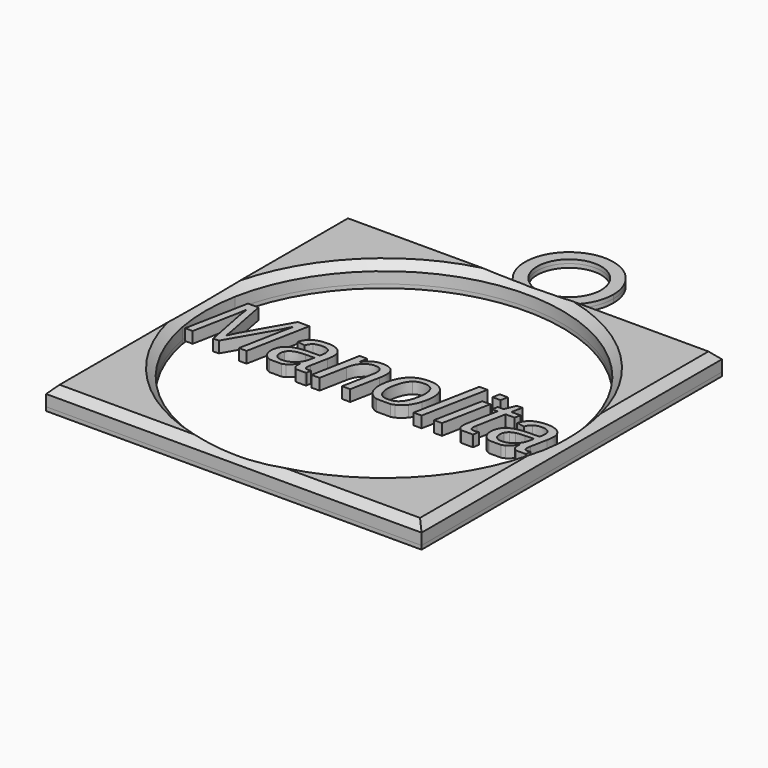
from build123d import *
from build123d import SkipClean  # not in build123d's __all__

# Parameters (mm, degrees)
F1_DEPTH     = 5
F0_R         = 8.5199022073
F2_DEPTH     = 1
F3_T1_DEPTH  = 58.7432495596
F3_T3_DEPTH  = 110.2867319519
F3_T5_DEPTH  = 110.2867319519
F3_T7_DEPTH  = 58.7432495596
F3_T10_ANGLE = 65.1626745713
F2_FACE_R    = 8.5199022073
F4_DEPTH     = 1
F5_DEPTH     = 3


# Not quite as in the source:
# - a fillet or chamfer that OpenCascade refuses, or shapes differently, is made with other operations: its cross-section is extruded or revolved along the edge and cut away or added
# - the program builds the solid bodies; features that only make, move or delete a surface that nothing else refers to are left out


with BuildPart() as f1:
    # F0 (on Top) → F1 (new body)
    with BuildSketch(Plane.XY):
        with BuildLine():
            Line((-50, 50), (-50, -50))
            Line((-50, -50), (50, -50))
            Line((50, -50), (50, 50))
            Line((50, 50), (1.5434823923, 50))
            ThreePointArc((1.5434823923, 50), (0, 49.898331828), (-1.5434823923, 50))
            Line((-1.5434823923, 50), (-50, 50))
        make_face()
        with BuildLine():
            ThreePointArc((46.6759421594, 8.8094508077), (47.2935368342, 4.4239545335), (47.5, 0))
            ThreePointArc((47.5, 0), (47.2935368342, -4.4239545335), (46.6759421594, -8.8094508077))
            ThreePointArc((46.6759421594, -8.8094508077), (0, -47.5), (-46.6759421594, -8.8094508077))
            ThreePointArc((-46.6759421594, -8.8094508077), (-47.5, 0), (-46.6759421594, 8.8094508077))
            ThreePointArc((-46.6759421594, 8.8094508077), (0, 47.5), (46.6759421594, 8.8094508077))
        make_face(mode=Mode.SUBTRACT)
    extrude(amount=F1_DEPTH)

    # F0 (on Top) → F2 (join)
    with BuildSketch(Plane.XY):
        with BuildLine():
            ThreePointArc((11.7670764853, 61.6654083133), (-7.7557015687, 70.5148818675), (-1.5434823923, 50))
            Line((-1.5434823923, 50), (1.5434823923, 50))
            ThreePointArc((1.5434823923, 50), (8.8494735542, 53.9097067445), (11.7670764853, 61.6654083133))
        make_face()
        with Locations((0, 61.6654083133)):
            Circle(F0_R, mode=Mode.SUBTRACT)
        with BuildLine():
            Line((-50, 50), (-50, -50))
            Line((-50, -50), (50, -50))
            Line((50, -50), (50, 50))
            Line((50, 50), (1.5434823923, 50))
            ThreePointArc((1.5434823923, 50), (0, 49.898331828), (-1.5434823923, 50))
            Line((-1.5434823923, 50), (-50, 50))
        make_face()
        with BuildLine():
            ThreePointArc((46.6759421594, 8.8094508077), (47.2935368342, 4.4239545335), (47.5, 0))
            ThreePointArc((47.5, 0), (47.2935368342, -4.4239545335), (46.6759421594, -8.8094508077))
            ThreePointArc((46.6759421594, -8.8094508077), (0, -47.5), (-46.6759421594, -8.8094508077))
            ThreePointArc((-46.6759421594, -8.8094508077), (-47.5, 0), (-46.6759421594, 8.8094508077))
            ThreePointArc((-46.6759421594, 8.8094508077), (0, 47.5), (46.6759421594, 8.8094508077))
        make_face(mode=Mode.SUBTRACT)
        with BuildLine():
            Line((1.5434823923, 50), (-1.5434823923, 50))
            ThreePointArc((-1.5434823923, 50), (0, 49.898331828), (1.5434823923, 50))
        make_face()
    extrude(amount=F2_DEPTH)

    # F3: chamfer of 2 on 7 edges, made by hand

    # F3_s2 → F3_t1 (cut)
    with BuildSketch(Plane.YZ.offset(-55.1433659759)):
        Polygon((48, 5), (50, 3), (50, 5), align=None)
    extrude(amount=F3_T1_DEPTH, mode=Mode.SUBTRACT)

    # F3_s4 → F3_t3 (cut)
    with BuildSketch(Plane.XZ.offset(-55.1433659759)):
        Polygon((-48, 5), (-50, 3), (-50, 5), align=None)
        Polygon((48, 5), (50, 3), (50, 5), align=None)
    extrude(amount=F3_T3_DEPTH, mode=Mode.SUBTRACT)

    # F3_s6 → F3_t5 (cut)
    with BuildSketch(Plane.YZ.offset(-55.1433659759)):
        Polygon((-48, 5), (-50, 3), (-50, 5), align=None)
    extrude(amount=F3_T5_DEPTH, mode=Mode.SUBTRACT)

    # F3_s8 → F3_t7 (cut)
    with BuildSketch(Plane.YZ.offset(-3.5998835836)):
        Polygon((48, 5), (50, 3), (50, 5), align=None)
    extrude(amount=F3_T7_DEPTH, mode=Mode.SUBTRACT)

    # F3_s9 → F3_t10 (revolve, cut)
    with BuildSketch(Plane(origin=(27.9808033762, 17.881631304, 0), x_dir=(0, 0, 1), z_dir=(0.8426278439, 0.5384963479, 0))):
        Polygon((3, -40.1939135628), (5, -38.1939135628), (5, -40.1939135628), align=None)
    revolve(axis=Axis((0, 61.6654083133, 5), (0, 0, -1)), revolution_arc=F3_T10_ANGLE, mode=Mode.SUBTRACT)

    # F3_s11 → F3_t12 (revolve, cut)
    with BuildSketch(Plane(origin=(0, 0, 0), x_dir=(0, 0, 1), z_dir=(0.1854621223, 0.9826514139, 0))):
        Polygon((5, -49.5), (3, -47.5), (5, -47.5), align=None)
    revolve(axis=Axis((0, 0, 5), (0, 0, 1)), mode=Mode.SUBTRACT)

    # F0 (on Top) + F2_face (on face) → F4 (join)
    with BuildSketch(Plane.XY):
        with BuildLine():
            Line((-50, 50), (-50, -50))
            Line((-50, -50), (50, -50))
            Line((50, -50), (50, 50))
            Line((50, 50), (1.5434823923, 50))
            ThreePointArc((1.5434823923, 50), (0, 49.898331828), (-1.5434823923, 50))
            Line((-1.5434823923, 50), (-50, 50))
        make_face()
        with BuildLine():
            ThreePointArc((46.6759421594, 8.8094508077), (47.2935368342, 4.4239545335), (47.5, 0))
            ThreePointArc((47.5, 0), (47.2935368342, -4.4239545335), (46.6759421594, -8.8094508077))
            ThreePointArc((46.6759421594, -8.8094508077), (0, -47.5), (-46.6759421594, -8.8094508077))
            ThreePointArc((-46.6759421594, -8.8094508077), (-47.5, 0), (-46.6759421594, 8.8094508077))
            ThreePointArc((-46.6759421594, 8.8094508077), (0, 47.5), (46.6759421594, 8.8094508077))
        make_face(mode=Mode.SUBTRACT)
        with BuildLine():
            ThreePointArc((11.7670764853, 61.6654083133), (-7.7557015687, 70.5148818675), (-1.5434823923, 50))
            Line((-1.5434823923, 50), (1.5434823923, 50))
            ThreePointArc((1.5434823923, 50), (8.8494735542, 53.9097067445), (11.7670764853, 61.6654083133))
        make_face()
        with Locations((0, 61.6654083133)):
            Circle(F0_R, mode=Mode.SUBTRACT)
        with BuildLine():
            Line((1.5434823923, 50), (-1.5434823923, 50))
            ThreePointArc((-1.5434823923, 50), (0, 49.898331828), (1.5434823923, 50))
        make_face()
    with BuildSketch(Plane(origin=(0, 61.6654083133, 1), x_dir=(1, 0, 0), z_dir=(0, 0, 1))):
        with BuildLine():
            ThreePointArc((-1.5434823923, -11.6654083133), (0, -11.7670764853), (1.5434823923, -11.6654083133))
            ThreePointArc((1.5434823923, -11.6654083133), (0, 11.7670764853), (-1.5434823923, -11.6654083133))
        make_face()
        Circle(F2_FACE_R, mode=Mode.SUBTRACT)
    with SkipClean():  # cleaning this boolean's faces spoils the solid; the shape is the same uncleaned
        extrude(amount=-F4_DEPTH)


with BuildPart() as f5:
    # F0 (on Top) → F5 (new body)
    with BuildSketch(Plane.XY):
        Polygon((25.5470249877, 6.8670892581), (25.9333310952, 8.8094508077), (23.7808877048, 8.8094508077), (23.3981919348, 6.8670892581), align=None)
        with BuildLine():
            Line((42.3061471078, -8.8094508077), (44.4772175829, -8.8094508077))
            add(Edge.make_bspline(
                [(44.8100515369, -8.7368034269), (44.6425976503, -8.7774475742), (44.4772175829, -8.8094508077)],
                knots=[0, 0, 0, 0.2125992126, 0.2125992126, 0.2125992126], degree=2))
            Line((44.8100515369, -8.7368034269), (44.9782875766, -7.3985622018))
            add(Edge.make_bspline(
                [(44.2594608614, -7.4826802217), (44.5844623018, -7.4826802217), (44.9782875766, -7.3985622018)],
                knots=[0, 0, 0, 1, 1, 1], degree=2))
            add(Edge.make_bspline(
                [(43.292103633, -6.6109116521), (43.292103633, -7.4826802217), (44.2594608614, -7.4826802217)],
                knots=[0, 0, 0, 1, 1, 1], degree=2))
            add(Edge.make_bspline(
                [(43.4221042091, -5.5594364038), (43.292103633, -6.1329683575), (43.292103633, -6.6109116521)],
                knots=[0, 0, 0, 1, 1, 1], degree=2))
            Line((43.4221042091, -5.5594364038), (44.3091669641, -1.0438281556))
            add(Edge.make_bspline(
                [(44.5347561992, 0.8335331059), (44.5347561992, 0.0688238344), (44.3091669641, -1.0438281556)],
                knots=[0, 0, 0, 1, 1, 1], degree=2))
            add(Edge.make_bspline(
                [(43.345633282, 3.4029562582), (44.5347561992, 2.4470696688), (44.5347561992, 0.8335331059)],
                knots=[0, 0, 0, 1, 1, 1], degree=2))
            add(Edge.make_bspline(
                [(40.1147366099, 4.3588428476), (42.1565103648, 4.3588428476), (43.345633282, 3.4029562582)],
                knots=[0, 0, 0, 1, 1, 1], degree=2))
            add(Edge.make_bspline(
                [(36.5339854461, 3.5635452052), (37.8664913517, 4.3588428476), (40.1147366099, 4.3588428476)],
                knots=[0, 0, 0, 1, 1, 1], degree=2))
            add(Edge.make_bspline(
                [(34.6661830504, 1.0132397847), (35.2014795405, 2.7682475628), (36.5339854461, 3.5635452052)],
                knots=[0, 0, 0, 1, 1, 1], degree=2))
            Line((34.6661830504, 1.0132397847), (36.7920748252, 0.6652970662))
            add(Edge.make_bspline(
                [(37.8435500735, 2.213833341), (37.1132527192, 1.7053016755), (36.7920748252, 0.6652970662)],
                knots=[0, 0, 0, 1, 1, 1], degree=2))
            add(Edge.make_bspline(
                [(39.9962066728, 2.7223650066), (38.5738474278, 2.7223650066), (37.8435500735, 2.213833341)],
                knots=[0, 0, 0, 1, 1, 1], degree=2))
            add(Edge.make_bspline(
                [(41.7512144509, 2.2023627019), (41.1165057556, 2.7223650066), (39.9962066728, 2.7223650066)],
                knots=[0, 0, 0, 1, 1, 1], degree=2))
            add(Edge.make_bspline(
                [(42.3859231463, 0.5926496854), (42.3859231463, 1.6823603973), (41.7512144509, 2.2023627019)],
                knots=[0, 0, 0, 1, 1, 1], degree=2))
            add(Edge.make_bspline(
                [(42.1565103648, -0.9214746722), (42.3859231463, 0.2485305132), (42.3859231463, 0.5926496854)],
                knots=[0, 0, 0, 1, 1, 1], degree=2))
            Line((42.1565103648, -0.9214746722), (39.3844392556, -0.9597101357))
            add(Edge.make_bspline(
                [(34.3373580637, -2.1411859602), (35.9203062557, -1.005592692), (39.3844392556, -0.9597101357)],
                knots=[0, 0, 0, 1, 1, 1], degree=2))
            add(Edge.make_bspline(
                [(32.7544098717, -5.486789023), (32.7544098717, -3.2767792284), (34.3373580637, -2.1411859602)],
                knots=[0, 0, 0, 1, 1, 1], degree=2))
            add(Edge.make_bspline(
                [(33.8001498004, -8.0447415362), (32.7544098717, -7.0391488442), (32.7544098717, -5.486789023)],
                knots=[0, 0, 0, 1, 1, 1], degree=2))
            add(Edge.make_bspline(
                [(35.0309562259, -8.8094508077), (34.3340710978, -8.558164941), (33.8001498004, -8.0447415362)],
                knots=[0.4894320446, 0.4894320446, 0.4894320446, 1, 1, 1], degree=2))
            Line((35.0309562259, -8.8094508077), (38.2424706133, -8.8094508077))
            add(Edge.make_bspline(
                [(39.0862026397, -8.4462139038), (38.6944582041, -8.6688600218), (38.2424706133, -8.8094508077)],
                knots=[0, 0, 0, 0.3685459817, 0.3685459817, 0.3685459817], degree=2))
            add(Edge.make_bspline(
                [(41.1432705801, -6.3356163144), (40.1491485271, -7.8420935793), (39.0862026397, -8.4462139038)],
                knots=[0, 0, 0, 1, 1, 1], degree=2))
            Line((41.1432705801, -6.3356163144), (41.2120944145, -6.3356163144))
            Line((41.2120944145, -6.3356163144), (41.1547412191, -7.1003255859))
            add(Edge.make_bspline(
                [(41.6613611115, -8.4691551819), (41.1547412191, -8.010329619), (41.1547412191, -7.1003255859)],
                knots=[0, 0, 0, 1, 1, 1], degree=2))
            add(Edge.make_bspline(
                [(42.3061471078, -8.8094508077), (41.9104838328, -8.6947757596), (41.6613611115, -8.4691551819)],
                knots=[0.5082650227, 0.5082650227, 0.5082650227, 1, 1, 1], degree=2))
        make_face()
        with BuildLine():
            Line((39.4914985536, -2.4508932152), (41.869744388, -2.4050106589))
            Line((41.869744388, -2.4050106589), (41.548566494, -3.9000172847))
            add(Edge.make_bspline(
                [(40.7475335321, -5.6187013724), (41.3573891761, -4.8176684105), (41.548566494, -3.9000172847)],
                knots=[0, 0, 0, 1, 1, 1], degree=2))
            add(Edge.make_bspline(
                [(39.20664435, -6.9148835876), (40.137677888, -6.4197343343), (40.7475335321, -5.6187013724)],
                knots=[0, 0, 0, 1, 1, 1], degree=2))
            add(Edge.make_bspline(
                [(37.1132527192, -7.4100328409), (38.2756108119, -7.4100328409), (39.20664435, -6.9148835876)],
                knots=[0, 0, 0, 1, 1, 1], degree=2))
            add(Edge.make_bspline(
                [(35.6163343203, -6.8498832995), (36.1956015934, -7.4100328409), (37.1132527192, -7.4100328409)],
                knots=[0, 0, 0, 1, 1, 1], degree=2))
            add(Edge.make_bspline(
                [(35.0370670471, -5.3912003641), (35.0370670471, -6.2897337581), (35.6163343203, -6.8498832995)],
                knots=[0, 0, 0, 1, 1, 1], degree=2))
            add(Edge.make_bspline(
                [(35.2932446531, -4.1313418393), (35.0370670471, -4.6494323707), (35.0370670471, -5.3912003641)],
                knots=[0, 0, 0, 1, 1, 1], degree=2))
            add(Edge.make_bspline(
                [(35.9967771828, -3.2710439089), (35.549422259, -3.6132513079), (35.2932446531, -4.1313418393)],
                knots=[0, 0, 0, 1, 1, 1], degree=2))
            add(Edge.make_bspline(
                [(37.2566357076, -2.7089825943), (36.4441321067, -2.9288365099), (35.9967771828, -3.2710439089)],
                knots=[0, 0, 0, 1, 1, 1], degree=2))
            add(Edge.make_bspline(
                [(39.4914985536, -2.4508932152), (38.0691393086, -2.4891286787), (37.2566357076, -2.7089825943)],
                knots=[0, 0, 0, 1, 1, 1], degree=2))
        make_face(mode=Mode.SUBTRACT)
        Polygon((20.4967286534, 8.8094508077), (18.3441462497, 8.8094508077), (14.9252132066, -8.8094508077), (17.0663991668, -8.8094508077), align=None)
        with BuildLine():
            Line((-42.661218484, 8.0256238044), (-45.922703527, -8.8094508077))
            Line((-45.922703527, -8.8094508077), (-43.8924004111, -8.8094508077))
            add(Edge.make_bspline(
                [(-41.5007721645, 3.6228101737), (-41.7512144509, 2.0991269503), (-43.8924004111, -8.8094508077)],
                knots=[0, 0, 0, 1, 1, 1], degree=2))
            add(Edge.make_bspline(
                [(-41.1432705801, 5.8653201124), (-41.2503298781, 5.1464933972), (-41.5007721645, 3.6228101737)],
                knots=[0, 0, 0, 1, 1, 1], degree=2))
            add(Edge.make_bspline(
                [(-40.6538566463, 2.5197170496), (-40.7265040271, 2.8638362218), (-41.1432705801, 5.8653201124)],
                knots=[0, 0, 0, 1, 1, 1], degree=2))
            Line((-40.6538566463, 2.5197170496), (-38.4438468517, -8.8094508077))
            Line((-38.4438468517, -8.8094508077), (-36.9603108649, -8.8094508077))
            Line((-36.9603108649, -8.8094508077), (-30.4143995009, 2.5197170496))
            add(Edge.make_bspline(
                [(-28.6823330009, 5.8653201124), (-29.7682201664, 3.6056042151), (-30.4143995009, 2.5197170496)],
                knots=[0, 0, 0, 1, 1, 1], degree=2))
            add(Edge.make_bspline(
                [(-29.4585129115, 2.2788336291), (-29.0264521731, 4.4888434237), (-28.6823330009, 5.8653201124)],
                knots=[0, 0, 0, 1, 1, 1], degree=2))
            Line((-29.4585129115, 2.2788336291), (-31.6073459644, -8.8094508077))
            Line((-31.6073459644, -8.8094508077), (-29.5541015704, -8.8094508077))
            Line((-29.5541015704, -8.8094508077), (-26.2926165275, 8.0256238044))
            Line((-26.2926165275, 8.0256238044), (-29.3514536135, 8.0256238044))
            Line((-29.3514536135, 8.0256238044), (-35.9585417193, -3.5520745661))
            Line((-35.9585417193, -3.5520745661), (-37.2011942855, -6.0985564402))
            add(Edge.make_bspline(
                [(-37.5835489212, -3.6476632251), (-37.4879602623, -4.1141358807), (-37.2011942855, -6.0985564402)],
                knots=[0, 0, 0, 1, 1, 1], degree=2))
            Line((-37.5835489212, -3.6476632251), (-39.8394412721, 8.0256238044))
            Line((-39.8394412721, 8.0256238044), (-42.661218484, 8.0256238044))
        make_face()
        with BuildLine():
            Line((5.021726883, -8.8094508077), (8.7657562591, -8.8094508077))
            add(Edge.make_bspline(
                [(9.7309254799, -8.4691551819), (9.2712635293, -8.6761733048), (8.7657562591, -8.8094508077)],
                knots=[0, 0, 0, 0.3562036935, 0.3562036935, 0.3562036935], degree=2))
            add(Edge.make_bspline(
                [(11.9103469037, -6.7237062697), (11.0213723755, -7.8879761356), (9.7309254799, -8.4691551819)],
                knots=[0, 0, 0, 1, 1, 1], degree=2))
            add(Edge.make_bspline(
                [(13.2772647265, -3.8808995529), (12.7993214318, -5.5594364038), (11.9103469037, -6.7237062697)],
                knots=[0, 0, 0, 1, 1, 1], degree=2))
            add(Edge.make_bspline(
                [(13.7552080212, -0.6500028808), (13.7552080212, -2.2023627019), (13.2772647265, -3.8808995529)],
                knots=[0, 0, 0, 1, 1, 1], degree=2))
            add(Edge.make_bspline(
                [(12.4303492083, 3.037807581), (13.7552080212, 1.7282429536), (13.7552080212, -0.6500028808)],
                knots=[0, 0, 0, 1, 1, 1], degree=2))
            add(Edge.make_bspline(
                [(8.5934204385, 4.3473722085), (11.1054903954, 4.3473722085), (12.4303492083, 3.037807581)],
                knots=[0, 0, 0, 1, 1, 1], degree=2))
            add(Edge.make_bspline(
                [(4.9247277085, 3.3781032069), (6.406351922, 4.3473722085), (8.5934204385, 4.3473722085)],
                knots=[0, 0, 0, 1, 1, 1], degree=2))
            add(Edge.make_bspline(
                [(2.6076586158, 0.5219140778), (3.4431034949, 2.4088342052), (4.9247277085, 3.3781032069)],
                knots=[0, 0, 0, 1, 1, 1], degree=2))
            add(Edge.make_bspline(
                [(1.7225076341, -3.8044286257), (1.7722137367, -1.3650060496), (2.6076586158, 0.5219140778)],
                knots=[0, 0, 0, 1, 1, 1], degree=2))
            add(Edge.make_bspline(
                [(3.0856019105, -7.6394456223), (1.7225076341, -6.2285570164), (1.7225076341, -3.8044286257)],
                knots=[0, 0, 0, 1, 1, 1], degree=2))
            add(Edge.make_bspline(
                [(5.021726883, -8.8094508077), (3.8854698095, -8.4673593803), (3.0856019105, -7.6394456223)],
                knots=[0.4131969353, 0.4131969353, 0.4131969353, 1, 1, 1], degree=2))
        make_face()
        with BuildLine():
            add(Edge.make_bspline(
                [(11.5337275874, -0.6500028808), (11.5337275874, 2.7682475628), (8.5704791604, 2.7682475628)],
                knots=[0, 0, 0, 1, 1, 1], degree=2))
            add(Edge.make_bspline(
                [(11.1207845808, -3.5157508757), (11.4725508457, -2.1526565993), (11.5337275874, -0.6500028808)],
                knots=[0, 0, 0, 1, 1, 1], degree=2))
            add(Edge.make_bspline(
                [(10.2069570014, -5.7563490412), (10.7690183159, -4.8788451522), (11.1207845808, -3.5157508757)],
                knots=[0, 0, 0, 1, 1, 1], degree=2))
            add(Edge.make_bspline(
                [(8.8993041471, -7.0467959369), (9.6448956868, -6.6338529303), (10.2069570014, -5.7563490412)],
                knots=[0, 0, 0, 1, 1, 1], degree=2))
            add(Edge.make_bspline(
                [(6.9225306803, -7.4597389435), (8.1537126074, -7.4597389435), (8.8993041471, -7.0467959369)],
                knots=[0, 0, 0, 1, 1, 1], degree=2))
            add(Edge.make_bspline(
                [(4.7010502466, -6.5325289518), (5.4657595181, -7.4597389435), (6.9225306803, -7.4597389435)],
                knots=[0, 0, 0, 1, 1, 1], degree=2))
            add(Edge.make_bspline(
                [(3.9363409751, -3.8388405429), (3.9363409751, -5.6053189601), (4.7010502466, -6.5325289518)],
                knots=[0, 0, 0, 1, 1, 1], degree=2))
            add(Edge.make_bspline(
                [(4.4735492383, -0.5754437268), (3.9363409751, -2.2597158973), (3.9363409751, -3.8388405429)],
                knots=[0, 0, 0, 1, 1, 1], degree=2))
            add(Edge.make_bspline(
                [(5.9838500495, 1.9385380033), (5.0107575015, 1.1088284437), (4.4735492383, -0.5754437268)],
                knots=[0, 0, 0, 1, 1, 1], degree=2))
            add(Edge.make_bspline(
                [(8.5704791604, 2.7682475628), (6.9569425975, 2.7682475628), (5.9838500495, 1.9385380033)],
                knots=[0, 0, 0, 1, 1, 1], degree=2))
        make_face(mode=Mode.SUBTRACT)
        Polygon((22.8705425375, 4.117959427), (20.362296127, -8.8094508077), (22.5034820872, -8.8094508077), (25.0231991368, 4.117959427), align=None)
        with BuildLine():
            Line((27.5877950428, -8.8094508077), (30.5493130455, -8.8094508077))
            add(Edge.make_bspline(
                [(30.758518673, -8.7597447051), (30.652735788, -8.785762502), (30.5493130455, -8.8094508077)],
                knots=[0, 0, 0, 0.089534532, 0.089534532, 0.089534532], degree=2))
            Line((30.758518673, -8.7597447051), (30.9841079081, -7.1729729667))
            add(Edge.make_bspline(
                [(29.7911614446, -7.3412090064), (30.2920460174, -7.3412090064), (30.9841079081, -7.1729729667)],
                knots=[0, 0, 0, 1, 1, 1], degree=2))
            add(Edge.make_bspline(
                [(28.7167449181, -6.2897337581), (28.7167449181, -7.3412090064), (29.7911614446, -7.3412090064)],
                knots=[0, 0, 0, 1, 1, 1], degree=2))
            add(Edge.make_bspline(
                [(28.8582161334, -5.1541404899), (28.7167449181, -5.8691436588), (28.7167449181, -6.2897337581)],
                knots=[0, 0, 0, 1, 1, 1], degree=2))
            Line((28.8582161334, -5.1541404899), (30.3532227591, 2.5541289668))
            Line((30.3532227591, 2.5541289668), (32.7429392326, 2.5541289668))
            Line((32.7429392326, 2.5541289668), (33.0526464876, 4.117959427))
            Line((33.0526464876, 4.117959427), (30.6629300141, 4.117959427))
            Line((30.6629300141, 4.117959427), (31.2249913287, 7.0123840197))
            Line((31.2249913287, 7.0123840197), (29.7911614446, 7.0123840197))
            Line((29.7911614446, 7.0123840197), (28.5370382393, 4.117959427))
            Line((28.5370382393, 4.117959427), (27.0190903354, 4.117959427))
            Line((27.0190903354, 4.117959427), (26.7093830804, 2.5541289668))
            Line((26.7093830804, 2.5541289668), (28.2005661599, 2.5541289668))
            Line((28.2005661599, 2.5541289668), (26.6979124414, -5.272670427))
            add(Edge.make_bspline(
                [(26.5182057626, -6.8250302482), (26.5182057626, -6.1673802747), (26.6979124414, -5.272670427)],
                knots=[0, 0, 0, 1, 1, 1], degree=2))
            add(Edge.make_bspline(
                [(27.0974730357, -8.4404785842), (26.5182057626, -7.8306229402), (26.5182057626, -6.8250302482)],
                knots=[0, 0, 0, 1, 1, 1], degree=2))
            add(Edge.make_bspline(
                [(27.5877950428, -8.8094508077), (27.3126836962, -8.667053504), (27.0974730357, -8.4404785842)],
                knots=[0.6284777848, 0.6284777848, 0.6284777848, 1, 1, 1], degree=2))
        make_face()
        with BuildLine():
            Line((-4.1160476539, -8.8094508077), (-1.9557439619, -8.8094508077))
            Line((-1.9557439619, -8.8094508077), (-0.4377960579, -1.005592692))
            add(Edge.make_bspline(
                [(-0.1854419983, 0.952063043), (-0.1854419983, 0.1873537715), (-0.4377960579, -1.005592692)],
                knots=[0, 0, 0, 1, 1, 1], degree=2))
            add(Edge.make_bspline(
                [(-1.0763282996, 3.4736918658), (-0.1854419983, 2.6000115231), (-0.1854419983, 0.952063043)],
                knots=[0, 0, 0, 1, 1, 1], degree=2))
            add(Edge.make_bspline(
                [(-3.7336930181, 4.3473722085), (-1.9672146009, 4.3473722085), (-1.0763282996, 3.4736918658)],
                knots=[0, 0, 0, 1, 1, 1], degree=2))
            add(Edge.make_bspline(
                [(-6.1081153061, 3.8158992648), (-5.1101697068, 4.3473722085), (-3.7336930181, 4.3473722085)],
                knots=[0, 0, 0, 1, 1, 1], degree=2))
            add(Edge.make_bspline(
                [(-8.096359412, 1.9079496324), (-7.1060609054, 3.2844263211), (-6.1081153061, 3.8158992648)],
                knots=[0, 0, 0, 1, 1, 1], degree=2))
            Line((-8.096359412, 1.9079496324), (-8.1307713293, 1.9079496324))
            add(Edge.make_bspline(
                [(-7.9223880528, 3.1926612085), (-8.0466533094, 2.3973635662), (-8.1307713293, 1.9079496324)],
                knots=[0, 0, 0, 1, 1, 1], degree=2))
            add(Edge.make_bspline(
                [(-7.7981227962, 4.117959427), (-7.7981227962, 3.9879588509), (-7.9223880528, 3.1926612085)],
                knots=[0, 0, 0, 1, 1, 1], degree=2))
            Line((-7.7981227962, 4.117959427), (-9.828425912, 4.117959427))
            add(Edge.make_bspline(
                [(-10.2948985676, 1.3573589569), (-10.0540151471, 2.4929522251), (-9.828425912, 4.117959427)],
                knots=[0, 0, 0, 1, 1, 1], degree=2))
            Line((-10.2948985676, 1.3573589569), (-12.2793191272, -8.8094508077))
            Line((-12.2793191272, -8.8094508077), (-10.1266625279, -8.8094508077))
            Line((-10.1266625279, -8.8094508077), (-8.715773922, -1.5676540066))
            add(Edge.make_bspline(
                [(-7.186355379, 1.5370656357), (-8.3334192862, 0.3900017285), (-8.715773922, -1.5676540066)],
                knots=[0, 0, 0, 1, 1, 1], degree=2))
            add(Edge.make_bspline(
                [(-4.5366377532, 2.684129543), (-6.0392914717, 2.684129543), (-7.186355379, 1.5370656357)],
                knots=[0, 0, 0, 1, 1, 1], degree=2))
            add(Edge.make_bspline(
                [(-2.395451793, 0.6882383444), (-2.395451793, 2.684129543), (-4.5366377532, 2.684129543)],
                knots=[0, 0, 0, 1, 1, 1], degree=2))
            add(Edge.make_bspline(
                [(-2.6133939354, -1.101181351), (-2.395451793, -0.0497061026), (-2.395451793, 0.6882383444)],
                knots=[0, 0, 0, 1, 1, 1], degree=2))
            Line((-2.6133939354, -1.101181351), (-4.1160476539, -8.8094508077))
        make_face()
        with BuildLine():
            add(Edge.make_bspline(
                [(-23.4654794978, -8.8094508077), (-24.1623646258, -8.558164941), (-24.6962859232, -8.0447415362)],
                knots=[0.4894320446, 0.4894320446, 0.4894320446, 1, 1, 1], degree=2))
            Line((-23.4654794978, -8.8094508077), (-20.2539651103, -8.8094508077))
            add(Edge.make_bspline(
                [(-19.4102330839, -8.4462139038), (-19.8019775195, -8.6688600218), (-20.2539651103, -8.8094508077)],
                knots=[0, 0, 0, 0.3685459817, 0.3685459817, 0.3685459817], degree=2))
            add(Edge.make_bspline(
                [(-17.3531651436, -6.3356163144), (-18.3472871965, -7.8420935793), (-19.4102330839, -8.4462139038)],
                knots=[0, 0, 0, 1, 1, 1], degree=2))
            Line((-17.3531651436, -6.3356163144), (-17.2843413092, -6.3356163144))
            Line((-17.2843413092, -6.3356163144), (-17.3416945045, -7.1003255859))
            add(Edge.make_bspline(
                [(-16.8350746121, -8.4691551819), (-17.3416945045, -8.010329619), (-17.3416945045, -7.1003255859)],
                knots=[0, 0, 0, 1, 1, 1], degree=2))
            add(Edge.make_bspline(
                [(-16.1902886159, -8.8094508077), (-16.5859518909, -8.6947757596), (-16.8350746121, -8.4691551819)],
                knots=[0.5082650227, 0.5082650227, 0.5082650227, 1, 1, 1], degree=2))
            Line((-16.1902886159, -8.8094508077), (-14.0192181408, -8.8094508077))
            add(Edge.make_bspline(
                [(-13.6863841867, -8.7368034269), (-13.8538380734, -8.7774475742), (-14.0192181408, -8.8094508077)],
                knots=[0, 0, 0, 0.2125992126, 0.2125992126, 0.2125992126], degree=2))
            Line((-13.6863841867, -8.7368034269), (-13.518148147, -7.3985622018))
            add(Edge.make_bspline(
                [(-14.2369748622, -7.4826802217), (-13.9119734218, -7.4826802217), (-13.518148147, -7.3985622018)],
                knots=[0, 0, 0, 1, 1, 1], degree=2))
            add(Edge.make_bspline(
                [(-15.2043320907, -6.6109116521), (-15.2043320907, -7.4826802217), (-14.2369748622, -7.4826802217)],
                knots=[0, 0, 0, 1, 1, 1], degree=2))
            add(Edge.make_bspline(
                [(-15.0743315145, -5.5594364038), (-15.2043320907, -6.1329683575), (-15.2043320907, -6.6109116521)],
                knots=[0, 0, 0, 1, 1, 1], degree=2))
            Line((-15.0743315145, -5.5594364038), (-14.1872687596, -1.0438281556))
            add(Edge.make_bspline(
                [(-13.9616795245, 0.8335331059), (-13.9616795245, 0.0688238344), (-14.1872687596, -1.0438281556)],
                knots=[0, 0, 0, 1, 1, 1], degree=2))
            add(Edge.make_bspline(
                [(-15.1508024417, 3.4029562582), (-13.9616795245, 2.4470696688), (-13.9616795245, 0.8335331059)],
                knots=[0, 0, 0, 1, 1, 1], degree=2))
            add(Edge.make_bspline(
                [(-18.3816991138, 4.3588428476), (-16.3399253588, 4.3588428476), (-15.1508024417, 3.4029562582)],
                knots=[0, 0, 0, 1, 1, 1], degree=2))
            add(Edge.make_bspline(
                [(-21.9624502776, 3.5635452052), (-20.629944372, 4.3588428476), (-18.3816991138, 4.3588428476)],
                knots=[0, 0, 0, 1, 1, 1], degree=2))
            add(Edge.make_bspline(
                [(-23.8302526732, 1.0132397847), (-23.2949561832, 2.7682475628), (-21.9624502776, 3.5635452052)],
                knots=[0, 0, 0, 1, 1, 1], degree=2))
            Line((-23.8302526732, 1.0132397847), (-21.7043608984, 0.6652970662))
            add(Edge.make_bspline(
                [(-20.6528856501, 2.213833341), (-21.3831830044, 1.7053016755), (-21.7043608984, 0.6652970662)],
                knots=[0, 0, 0, 1, 1, 1], degree=2))
            add(Edge.make_bspline(
                [(-18.5002290508, 2.7223650066), (-19.9225882958, 2.7223650066), (-20.6528856501, 2.213833341)],
                knots=[0, 0, 0, 1, 1, 1], degree=2))
            add(Edge.make_bspline(
                [(-16.7452212727, 2.2023627019), (-17.3799299681, 2.7223650066), (-18.5002290508, 2.7223650066)],
                knots=[0, 0, 0, 1, 1, 1], degree=2))
            add(Edge.make_bspline(
                [(-16.1105125774, 0.5926496854), (-16.1105125774, 1.6823603973), (-16.7452212727, 2.2023627019)],
                knots=[0, 0, 0, 1, 1, 1], degree=2))
            add(Edge.make_bspline(
                [(-16.3399253588, -0.9214746722), (-16.1105125774, 0.2485305132), (-16.1105125774, 0.5926496854)],
                knots=[0, 0, 0, 1, 1, 1], degree=2))
            Line((-16.3399253588, -0.9214746722), (-19.111996468, -0.9597101357))
            add(Edge.make_bspline(
                [(-24.15907766, -2.1411859602), (-22.576129468, -1.005592692), (-19.111996468, -0.9597101357)],
                knots=[0, 0, 0, 1, 1, 1], degree=2))
            add(Edge.make_bspline(
                [(-25.742025852, -5.486789023), (-25.742025852, -3.2767792284), (-24.15907766, -2.1411859602)],
                knots=[0, 0, 0, 1, 1, 1], degree=2))
            add(Edge.make_bspline(
                [(-24.6962859232, -8.0447415362), (-25.742025852, -7.0391488442), (-25.742025852, -5.486789023)],
                knots=[0, 0, 0, 1, 1, 1], degree=2))
        make_face()
        with BuildLine():
            Line((-19.00493717, -2.4508932152), (-16.6266913357, -2.4050106589))
            Line((-16.6266913357, -2.4050106589), (-16.9478692297, -3.9000172847))
            add(Edge.make_bspline(
                [(-17.7489021916, -5.6187013724), (-17.1390465476, -4.8176684105), (-16.9478692297, -3.9000172847)],
                knots=[0, 0, 0, 1, 1, 1], degree=2))
            add(Edge.make_bspline(
                [(-19.2897913737, -6.9148835876), (-18.3587578356, -6.4197343343), (-17.7489021916, -5.6187013724)],
                knots=[0, 0, 0, 1, 1, 1], degree=2))
            add(Edge.make_bspline(
                [(-21.3831830044, -7.4100328409), (-20.2208249117, -7.4100328409), (-19.2897913737, -6.9148835876)],
                knots=[0, 0, 0, 1, 1, 1], degree=2))
            add(Edge.make_bspline(
                [(-22.8801014034, -6.8498832995), (-22.3008341302, -7.4100328409), (-21.3831830044, -7.4100328409)],
                knots=[0, 0, 0, 1, 1, 1], degree=2))
            add(Edge.make_bspline(
                [(-23.4593686765, -5.3912003641), (-23.4593686765, -6.2897337581), (-22.8801014034, -6.8498832995)],
                knots=[0, 0, 0, 1, 1, 1], degree=2))
            add(Edge.make_bspline(
                [(-23.2031910706, -4.1313418393), (-23.4593686765, -4.6494323707), (-23.4593686765, -5.3912003641)],
                knots=[0, 0, 0, 1, 1, 1], degree=2))
            add(Edge.make_bspline(
                [(-22.4996585408, -3.2710439089), (-22.9470134646, -3.6132513079), (-23.2031910706, -4.1313418393)],
                knots=[0, 0, 0, 1, 1, 1], degree=2))
            add(Edge.make_bspline(
                [(-21.239800016, -2.7089825943), (-22.052303617, -2.9288365099), (-22.4996585408, -3.2710439089)],
                knots=[0, 0, 0, 1, 1, 1], degree=2))
            add(Edge.make_bspline(
                [(-19.00493717, -2.4508932152), (-20.427296415, -2.4891286787), (-21.239800016, -2.7089825943)],
                knots=[0, 0, 0, 1, 1, 1], degree=2))
        make_face(mode=Mode.SUBTRACT)
    extrude(amount=F5_DEPTH)


solid = Compound([f1.part, f5.part])
